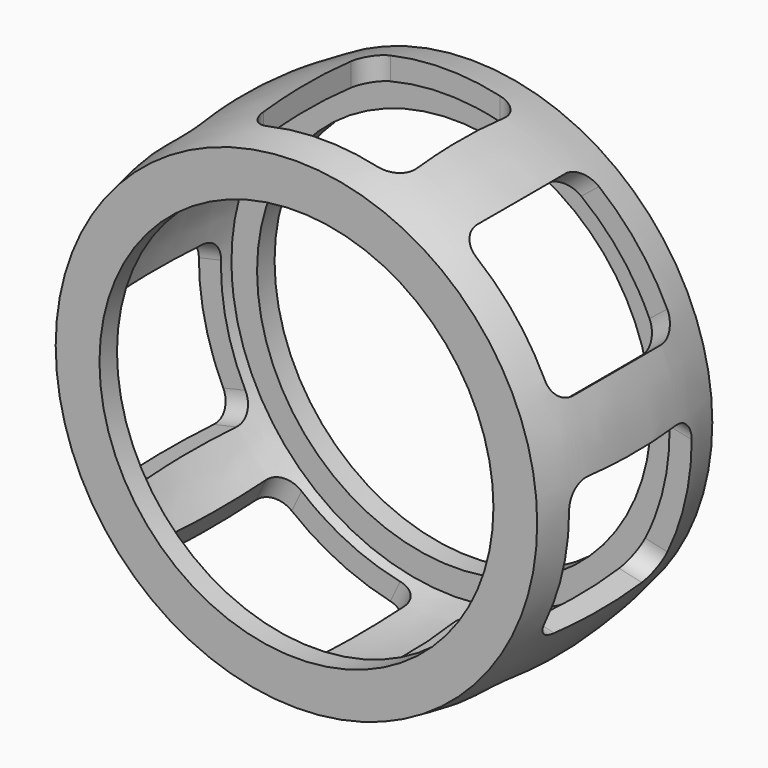
from build123d import *

# Parameters (mm, degrees)
F2_T            = -1
F4_DEPTH        = 11.5061026722
F4_COPIES_COUNT = 7


# Not quite as in the source:
# - a pattern or mirror of a feature is missing from the dataset's text; its kind, count and spacing are read off the source's solid


with BuildPart() as f1:
    # F0 (on Top) → F1 (revolve)
    with BuildSketch(Plane.XY):
        with BuildLine():
            Line((-9, -5), (-9, 5))
            Line((-9, 5), (-11, 5))
            ThreePointArc((-11, 5), (-11.5051025722, 0), (-11, -5))
            Line((-11, -5), (-9, -5))
        make_face()
    revolve(axis=Axis((0, -6.6258087754, 0), (0, -1, 0)))

    # F2
    f2_openings = [f1.faces().sort_by_distance(p)[0] for p in [
        (9, 0, 0),
    ]]
    offset(amount=F2_T, openings=f2_openings, kind=Kind.INTERSECTION)

    # F3 (on Top) → F4 (cut, through all)
    with BuildSketch(Plane.XY):
        with BuildLine():
            Line((2.5, 3.5), (-2.5, 3.5))
            ThreePointArc((-2.5, 3.5), (-3.2071067812, 3.2071067812), (-3.5, 2.5))
            Line((-3.5, 2.5), (-3.5, -2.5))
            ThreePointArc((-3.5, -2.5), (-3.2071067812, -3.2071067812), (-2.5, -3.5))
            Line((-2.5, -3.5), (2.5, -3.5))
            ThreePointArc((2.5, -3.5), (3.2071067812, -3.2071067812), (3.5, -2.5))
            Line((3.5, -2.5), (3.5, 2.5))
            ThreePointArc((3.5, 2.5), (3.2071067812, 3.2071067812), (2.5, 3.5))
        make_face()
    f4 = extrude(amount=F4_DEPTH, mode=Mode.SUBTRACT)

    # F4_copies: F4 ×7 about axis
    f4_copies_axis = Axis((0, 0, 0), (0, 1, 0))
    for i in range(1, F4_COPIES_COUNT):
        add(f4.rotate(f4_copies_axis, i * 360 / F4_COPIES_COUNT), mode=Mode.SUBTRACT)


solid = f1.part
